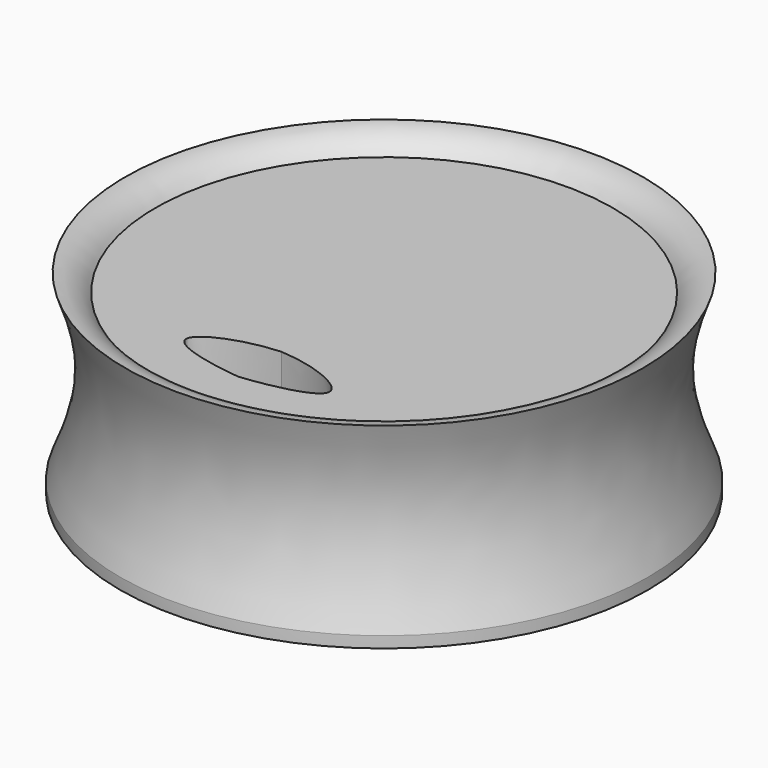
from build123d import *

# Parameters (mm, degrees)
F0_R     = 38.1
F0_R_2   = 33.02
F1_DEPTH = 27.94
F2_DEPTH = 25.4


# Not quite as in the source:
# - a fillet or chamfer that OpenCascade refuses, or shapes differently, is made with other operations: its cross-section is extruded or revolved along the edge and cut away or added


with BuildPart() as f1:
    # F0 (on Top) → F1 (new body)
    with BuildSketch(Plane.XY):
        Circle(F0_R)
        Circle(F0_R_2, mode=Mode.SUBTRACT)
    extrude(amount=F1_DEPTH)

    # F0 (on Top) → F2 (join)
    with BuildSketch(Plane.XY):
        Circle(F0_R_2)
        with BuildLine():
            add(Edge.make_bspline(
                [(0, -18.5258053243), (-5.2355541848, -18.7942963094), (-15.57457148, -23.313863117), (-4.9670636654, -25.775032118), (0, -26.312014088)],
                knots=[0, 0, 0, 0, 0.5032090963, 1, 1, 1, 1], degree=3))
            add(Edge.make_bspline(
                [(0, -18.5258053243), (5.2355541848, -18.7942963094), (15.57457148, -23.313863117), (4.9670636654, -25.775032118), (0, -26.312014088)],
                knots=[0, 0, 0, 0, 0.5032090963, 1, 1, 1, 1], degree=3))
        make_face(mode=Mode.SUBTRACT)
    extrude(amount=F2_DEPTH)

    # F3: fillet of radius 5.588 on 1 edges, made by hand

    # F3_s1 → F3_t2 (revolve, cut)
    with BuildSketch(Plane.XZ):
        with BuildLine():
            ThreePointArc((37.7035285843, 27.94), (35.03955411, 27.2641262199), (33.02, 25.4))
            Line((33.02, 25.4), (32.9263294283, 25.46096))
            ThreePointArc((32.9263294283, 25.46096), (32.90824, 26.67), (32.90824, 27.94))
            Line((32.90824, 27.94), (33.02, 28.05176))
            Line((33.02, 28.05176), (37.7035285843, 28.05176))
            Line((37.7035285843, 28.05176), (37.7035285843, 27.94))
        make_face()
    revolve(axis=Axis((0, 0, 27.94), (0, 0, 1)), mode=Mode.SUBTRACT)

    # F4 (on Front) → F5 (revolve, cut)
    with BuildSketch(Plane.XZ):
        with BuildLine():
            Line((38.7967936695, 0), (38.3886620402, 30.4337646812))
            add(Edge.make_bspline(
                [(38.3886620402, 30.4337646812), (33.1585071981, 18.5258053243), (33.9639782906, 11.0080875456), (38.7967936695, 0)],
                knots=[0, 0, 0, 0, 30.4365011803, 30.4365011803, 30.4365011803, 30.4365011803], degree=3))
        make_face()
    revolve(axis=Axis((0, 0, 6.5780002624), (0, 0, -1)), mode=Mode.SUBTRACT)


solid = f1.part
